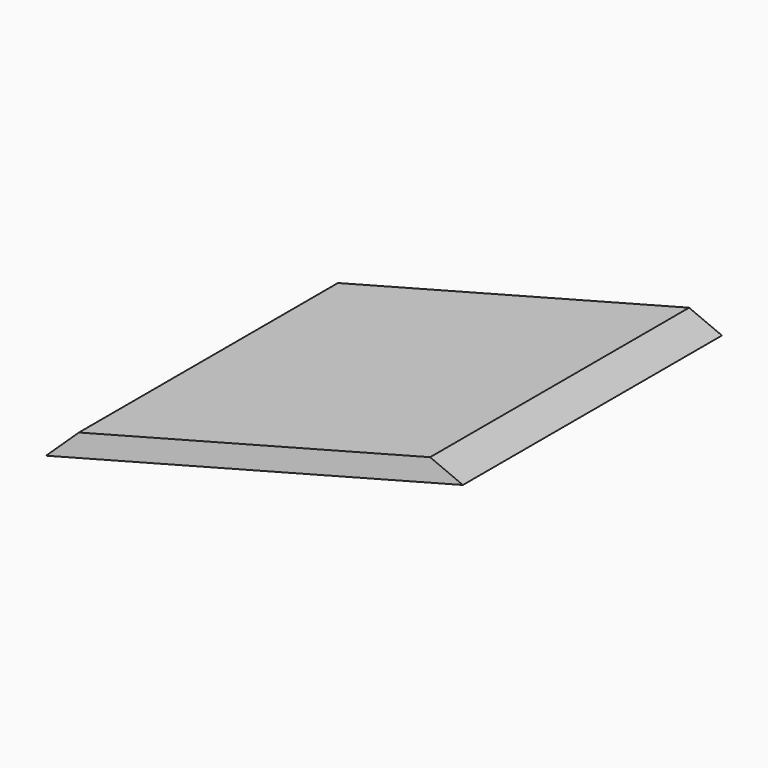
from build123d import *

# Parameters (mm, degrees)
F1_DEPTH = 19.05
F2_SIZE  = 19.04999
F3_SIZE  = 19.04999


# Not quite as in the source:
# - a fillet or chamfer is up to 0.001 mm smaller than in the source, because OpenCascade refuses the exact size


with BuildPart() as f1:
    # F0 (on Top) → F1 (new body)
    with BuildSketch(Plane.XY):
        Polygon((-120.9837489087, -207.2259), (120.9837489087, -67.5259), (120.9837489087, 207.2259), (-120.9837489087, 67.5259), align=None)
    extrude(amount=F1_DEPTH)

    # F2 (size 19.05 in the source; OpenCascade refuses exactly that, so slightly less here)
    f2_edges = [f1.edges().sort_by_distance(p)[0] for p in [
        (-120.983749, -69.85, 19.05),
    ]]
    chamfer(f2_edges, length=F2_SIZE)

    # F3 (size 19.05 in the source; OpenCascade refuses exactly that, so slightly less here)
    f3_edges = [f1.edges().sort_by_distance(p)[0] for p in [
        (120.983749, 69.85, 19.05),
    ]]
    chamfer(f3_edges, length=F3_SIZE)


solid = f1.part
